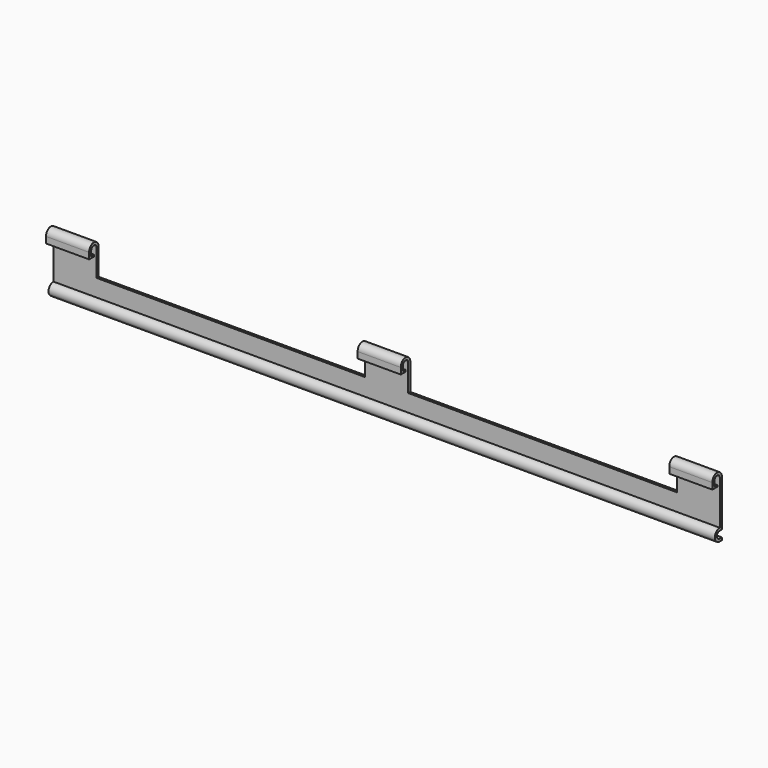
from build123d import *

# Parameters (mm, degrees)
F1_DEPTH      = 193.3
F2_W          = 155.8
F2_H          = 27.6261721705
F2_H_2        = 29.0520395572
F3_DEPTH      = 392
F3_DEPTH_BACK = 6.9075074824


# Not quite as in the source:
# - an extrude ends at something that could not be found from the text; its depth is read off the source's solid


with BuildPart() as f1:
    # F0 (on Right) → F1 (new body, symmetric)
    with BuildSketch(Plane.YZ):
        with BuildLine():
            Line((0, -17.0077651882), (0, -15.5077651882))
            Line((0, -15.5077651882), (-1.6385802936, -15.5077651882))
            ThreePointArc((-1.6385802936, -15.5077651882), (-3.6361192163, -13.605291718), (-1.8332301129, -11.5174320644))
            Line((-1.8332301129, -11.5174320644), (0, -11.5174320644))
            Line((0, -11.5174320644), (0, 15.5389810706))
            ThreePointArc((0, 15.5389810706), (-3.59937308, 18.9891420146), (-6.8941418337, 15.2470041272))
            Line((-6.8941418337, 15.2470041272), (-6.8941418337, 11.6459712901))
            Line((-6.8941418337, 11.6459712901), (-3.368163947, 11.6459712901))
            Line((-3.368163947, 11.6459712901), (-3.368163947, 12.6215412629))
            Line((-3.368163947, 12.6215412629), (-5.4103266448, 12.6215412629))
            Line((-5.4103266448, 12.6215412629), (-5.4103266448, 15.5389810706))
            ThreePointArc((-5.4103266448, 15.5389810706), (-3.5143862992, 17.4950989506), (-1.5, 15.661186523))
            Line((-1.5, 15.661186523), (-1.5, -10.0106816226))
            ThreePointArc((-1.5, -10.0106816226), (-5.1378081699, -13.4385473486), (-1.6385802936, -17.0077651882))
            Line((-1.6385802936, -17.0077651882), (0, -17.0077651882))
        make_face()
    extrude(amount=F1_DEPTH, both=True)

    # F2 (on Front) → F3 (cut, two sides)
    with BuildSketch(Plane.XZ) as f3_sk:
        with Locations((-90.4, 13.8130860853)):
            Rectangle(F2_W, F2_H)
        with Locations((90.4, 14.5260197786)):
            Rectangle(F2_W, F2_H_2)
    extrude(amount=-F3_DEPTH, mode=Mode.SUBTRACT)
    extrude(f3_sk.sketch, amount=F3_DEPTH_BACK, mode=Mode.SUBTRACT)


solid = f1.part
